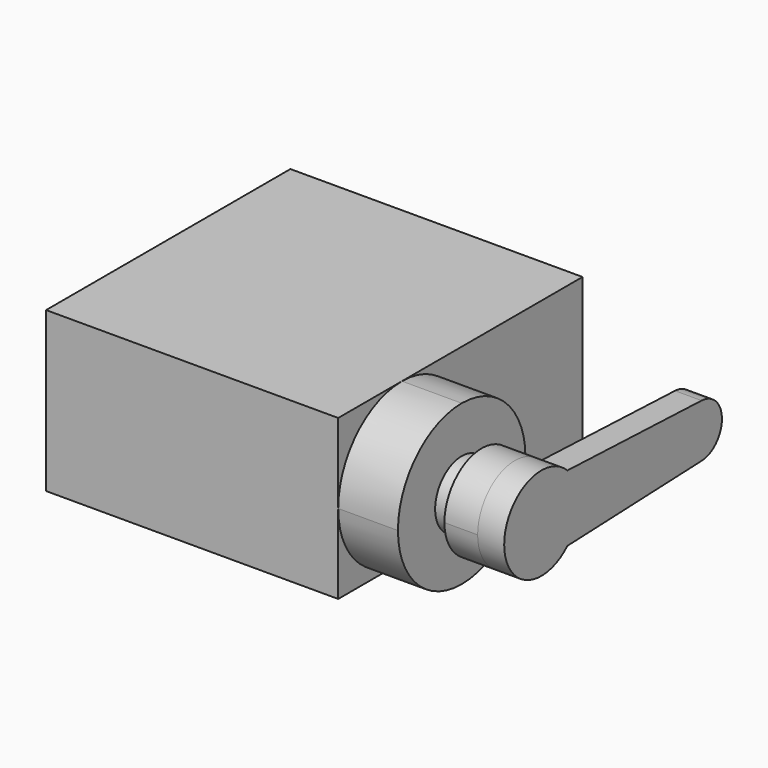
from build123d import *
from build123d import SkipClean  # not in build123d's __all__

# Parameters (mm, degrees)
F0_W     = 23
F0_H     = 12
F1_DEPTH = 22
F3_DEPTH = 4.5
F4_R     = 2.5
F5_DEPTH = 4
F6_R     = 2.5
F7_DEPTH = 2
F8_R     = 2.5
F9_DEPTH = 2.5


with BuildPart() as f1:
    # F0 (on Right) → F1 (new body)
    with BuildSketch(Plane.YZ):
        Rectangle(F0_W, F0_H)
    extrude(amount=F1_DEPTH)

    # F2 (on face) → F3 (join)
    with BuildSketch(Plane.YZ.offset(22)):
        with BuildLine():
            ThreePointArc((-5.5, -6), (-1.2573593129, -4.2426406871), (0.5, 0))
            ThreePointArc((0.5, 0), (-1.2573593129, 4.2426406871), (-5.5, 6))
            ThreePointArc((-5.5, 6), (-9.7426406871, 4.2426406871), (-11.5, 0))
            ThreePointArc((-11.5, 0), (-9.7426406871, -4.2426406871), (-5.5, -6))
        make_face()
    extrude(amount=F3_DEPTH)

    # F4 (on face) → F5 (join)
    with BuildSketch(Plane.YZ.offset(26.5)):
        with Locations((-5.5, 0)):
            Circle(F4_R)
    extrude(amount=F5_DEPTH)

    # F6 (on face) → F7 (join)
    with BuildSketch(Plane.YZ.offset(30.5)):
        with BuildLine():
            Line((-3.0505102572, -2.5), (9.5793642451, -1.9984247088))
            ThreePointArc((9.5793642451, -1.9984247088), (11.5, 0), (9.5793642451, 1.9984247088))
            Line((9.5793642451, 1.9984247088), (-3.0505102572, 2.5))
            ThreePointArc((-3.0505102572, 2.5), (-9, 0), (-3.0505102572, -2.5))
        make_face()
        with Locations((-5.5, 0)):
            Circle(F6_R, mode=Mode.SUBTRACT)
        with Locations((-5.5, 0)):
            Circle(F6_R)
    extrude(amount=F7_DEPTH)

    # F8 (on face) → F9 (join)
    with BuildSketch(Plane(origin=(30.5, 0, 0), x_dir=(0, -1, 0), z_dir=(-1, 0, 0))):
        with BuildLine():
            ThreePointArc((3.0505102572, -2.5), (6.8558735008, -3.2267021942), (9, 0))
            ThreePointArc((9, 0), (6.8558735008, 3.2267021942), (3.0505102572, 2.5))
            ThreePointArc((3.0505102572, 2.5), (2, 0), (3.0505102572, -2.5))
        make_face()
        with Locations((5.5, 0)):
            Circle(F8_R, mode=Mode.SUBTRACT)
    with SkipClean():  # cleaning this boolean's faces spoils the solid; the shape is the same uncleaned
        extrude(amount=F9_DEPTH)


solid = f1.part
